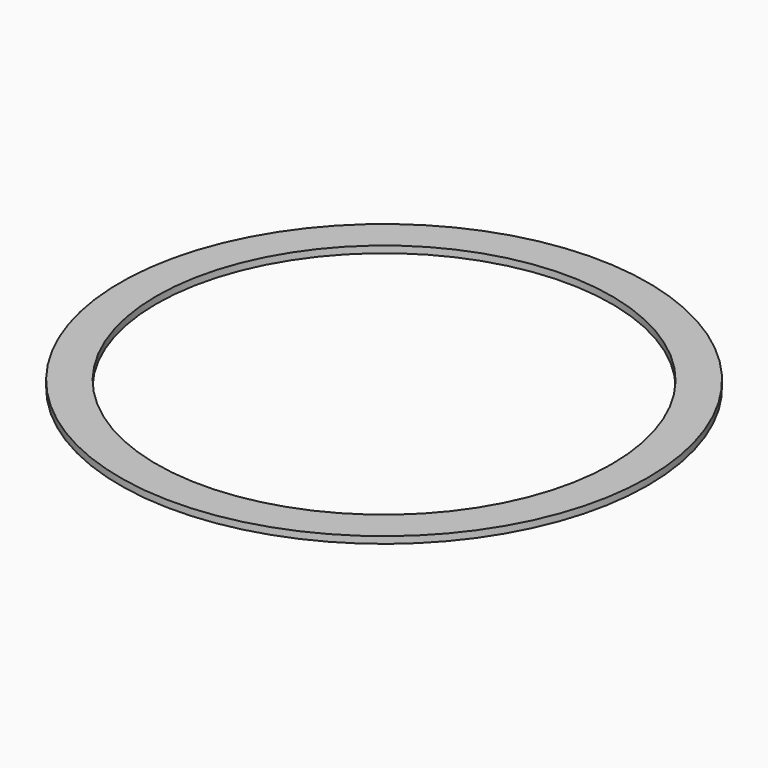
from build123d import *

# Parameters (mm, degrees)
F0_R     = 184.5691
F0_R_2   = 159.1691
F1_DEPTH = 4.7625


# Not quite as in the source:
# - a length typed as a fraction of an inch, garbled in the dataset ("3 / 203.2 mm" for 3/8 in), is restored


with BuildPart() as f1:
    # F0 (on Top) → F1 (new body)
    with BuildSketch(Plane.XY):
        Circle(F0_R)
        Circle(F0_R_2, mode=Mode.SUBTRACT)
    extrude(amount=F1_DEPTH)


solid = f1.part
